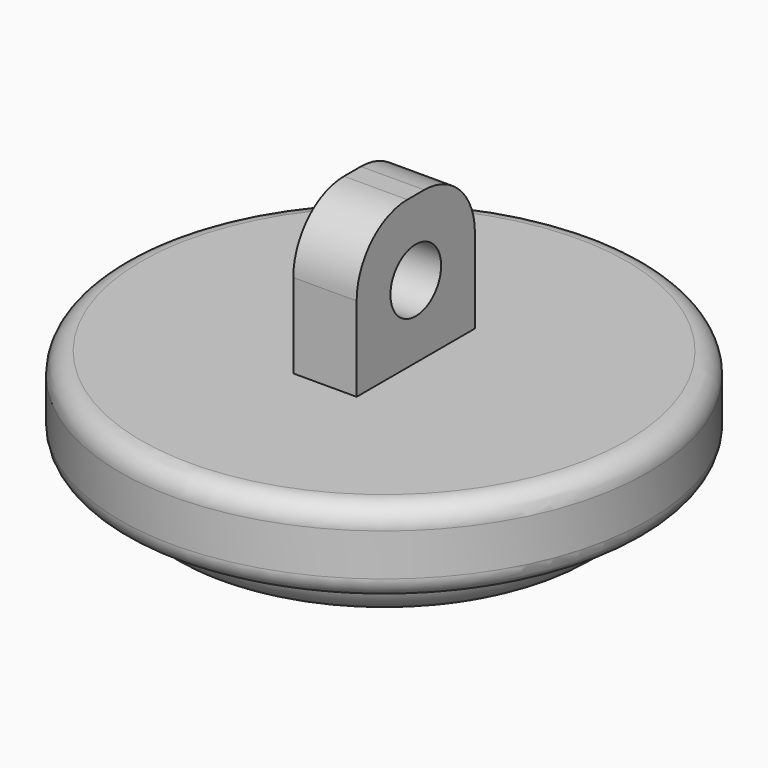
from build123d import *

# Parameters (mm, degrees)
F0_R     = 10.5
F1_DEPTH = 2
F0_R_2   = 12.5
F2_DEPTH = 4
F3_W     = 3
F3_H     = 7
F4_DEPTH = 7
F6_R     = 3
F5_R     = 1.5
F7_DEPTH = 25
F8_R     = 1.99999
F9_R     = 1


# Not quite as in the source:
# - a fillet or chamfer is up to 0.001 mm smaller than in the source, because OpenCascade refuses the exact size


with BuildPart() as f1:
    # F0 (on Top) → F1 (new body)
    with BuildSketch(Plane.XY):
        Circle(F0_R)
    extrude(amount=-F1_DEPTH)

    # F0 (on Top) → F2 (join)
    with BuildSketch(Plane.XY):
        Circle(F0_R_2)
        Circle(F0_R, mode=Mode.SUBTRACT)
        Circle(F0_R)
    extrude(amount=F2_DEPTH)

    # F3 (on face) → F4 (join)
    with BuildSketch(Plane.XY.offset(4)):
        Rectangle(F3_W, F3_H)
    extrude(amount=F4_DEPTH)

    # F6
    f6_edges = [f1.edges().sort_by_distance(p)[0] for p in [
        (0, -3.5, 11),
        (0, 3.5, 11),
    ]]
    fillet(f6_edges, radius=F6_R)

    # F5 (on face) → F7 (cut)
    with BuildSketch(Plane.YZ.offset(1.5)):
        with Locations((0, 7.438564696)):
            Circle(F5_R)
    extrude(amount=-F7_DEPTH, mode=Mode.SUBTRACT)

    # F8 (radius 2 in the source; OpenCascade refuses exactly that, so slightly less here)
    f8_edges = [f1.edges().sort_by_distance(p)[0] for p in [
        (-10.5, 0, -2),
    ]]
    fillet(f8_edges, radius=F8_R)

    # F9
    f9_edges = [f1.edges().sort_by_distance(p)[0] for p in [
        (12.5, 0, 2),
        (-12.5, 0, 0),
        (-12.5, 0, 4),
    ]]
    fillet(f9_edges, radius=F9_R)


solid = f1.part
